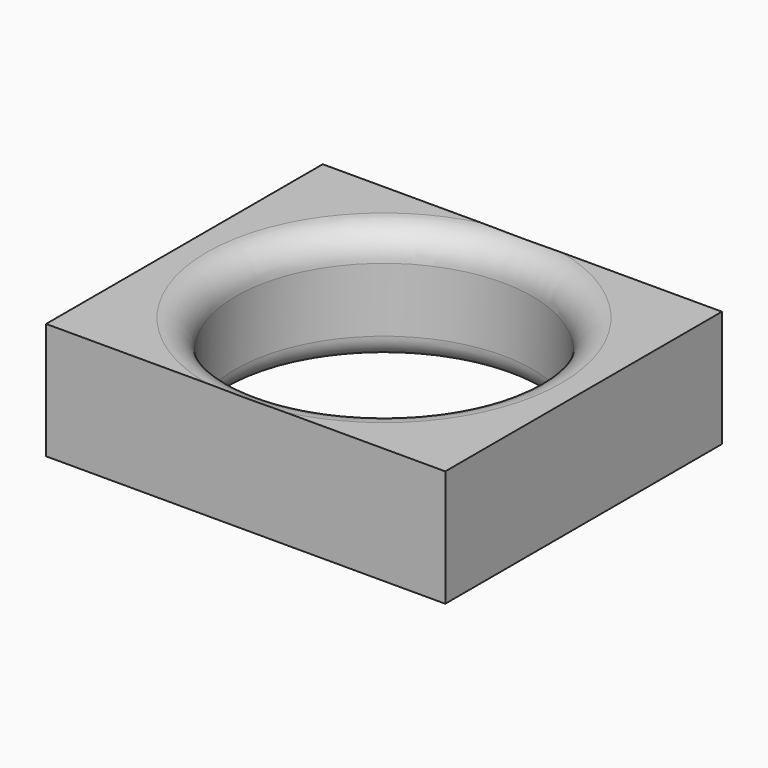
from build123d import *

# Parameters (mm, degrees)
F0_W     = 86.9801938534
F0_H     = 75.3522887826
F0_R     = 32.2813153837
F1_DEPTH = 25.4
F3_R     = 5.08


# Not quite as in the source:
# - a fillet or chamfer that OpenCascade refuses, or shapes differently, is made with other operations: its cross-section is extruded or revolved along the edge and cut away or added


with BuildPart() as f1:
    # F0 (on Top) → F1 (new body)
    with BuildSketch(Plane.XY):
        with Locations((13.0896866322, -5.9322379529)):
            Rectangle(F0_W, F0_H)
        with Locations((13.0896866322, -5.9322379529)):
            Circle(F0_R, mode=Mode.SUBTRACT)
    extrude(amount=F1_DEPTH)

    # F2: fillet of radius 6.35 on 1 edges, made by hand

    # F2_s1 → F2_t2 (revolve, cut)
    with BuildSketch(Plane.XZ.offset(5.9322379529)):
        with BuildLine():
            ThreePointArc((45.3710020159, 19.05), (47.2308739553, 23.5401280605), (51.7210020159, 25.4))
            Line((51.7210020159, 25.4), (45.3710020159, 25.4))
            Line((45.3710020159, 25.4), (45.3710020159, 19.05))
        make_face()
    revolve(axis=Axis((13.0896866322, -5.9322379529, 25.4), (0, 0, 1)), mode=Mode.SUBTRACT)

    # F3
    f3_edges = [f1.edges().sort_by_distance(p)[0] for p in [
        (-19.191629, -5.932238, 0),
    ]]
    fillet(f3_edges, radius=F3_R)


solid = f1.part
